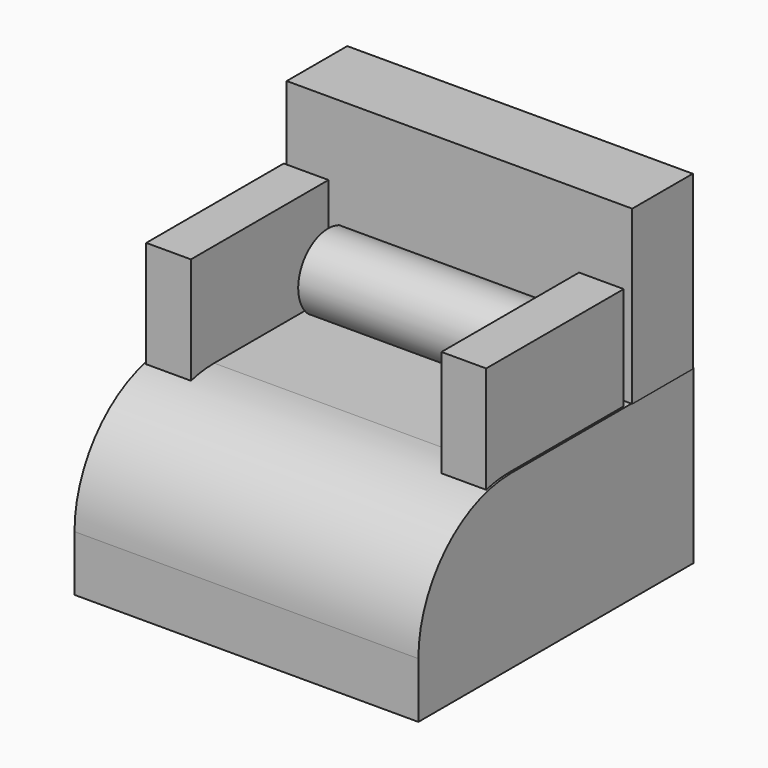
from build123d import *

# Parameters (mm, degrees)
F0_W          = 100
F0_H          = 100
F1_DEPTH      = 50
F4_DEPTH      = 50
F5_W          = 13
F5_H          = 50
F6_DEPTH      = 30
F8_R          = 10.8467438632
F9_DEPTH      = 35
F10_T4_DEPTH  = 268.9949493661
F10_T9_DEPTH  = 268.9949493661
F10_T14_DEPTH = 268.9949493661
F10_T20_DEPTH = 268.9949493661


# Not quite as in the source:
# - a fillet or chamfer that OpenCascade refuses, or shapes differently, is made with other operations: its cross-section is extruded or revolved along the edge and cut away or added


with BuildPart() as f1:
    # F0 (on Top) → F1 (new body)
    with BuildSketch(Plane.XY):
        Rectangle(F0_W, F0_H)
    extrude(amount=F1_DEPTH)

    # F3 (on offset) → F4 (join)
    with BuildSketch(Plane.XY.offset(50)):
        Polygon((49.7613176703, 49.4384859949), (-50.2386823297, 49.4384859949), (-50.2386823297, 27.4384859949), (-42.6304154098, 27.4384859949), (49.7613176703, 27.4384859949), align=None)
    extrude(amount=F4_DEPTH)

    # F5 (on offset) → F6 (join)
    with BuildSketch(Plane.XY.offset(50)):
        with Locations((-42.9296287298, 0.3518681973)):
            Rectangle(F5_W, F5_H)
    extrude(amount=F6_DEPTH)

    # F7: F1 across plane


with BuildPart() as f1_1:
    add(f1.part)
    add(f1.part.mirror(Plane.YZ))

    # F8 (on Right) → F9 (join, symmetric)
    with BuildSketch(Plane.YZ):
        with Locations((23.399380967, 57.991553098)):
            Circle(F8_R)
    extrude(amount=F9_DEPTH, both=True)

    # F10: fillet of radius 33.7989898732 on 1 edges, made by hand


with BuildPart() as f10_tool2:
    # F10_s3 → F10_t4 (new body)
    with BuildSketch(Plane.YZ.offset(-134.4974746831)):
        with BuildLine():
            ThreePointArc((-50, 16.2010101268), (-40.1005050634, 40.1005050634), (-16.2010101268, 50))
            Line((-16.2010101268, 50), (-50, 50))
            Line((-50, 50), (-50, 16.2010101268))
        make_face()
    extrude(amount=F10_T4_DEPTH)

    split(bisect_by=Plane.XZ.offset(24.6481318027), keep=Keep.TOP)


with BuildPart() as f1_2:
    add(f1_1.part)

    # F10_t1: cut F10_tool2
    add(f10_tool2.part, mode=Mode.SUBTRACT)


with BuildPart() as f10_tool7:
    # F10_s8 → F10_t9 (new body)
    with BuildSketch(Plane.YZ.offset(-134.4974746831)):
        with BuildLine():
            ThreePointArc((-50, 16.2010101268), (-40.1005050634, 40.1005050634), (-16.2010101268, 50))
            Line((-16.2010101268, 50), (-50, 50))
            Line((-50, 50), (-50, 16.2010101268))
        make_face()
    extrude(amount=F10_T9_DEPTH)

    split(bisect_by=Plane.YZ.offset(-49.4296287298), keep=Keep.BOTTOM)


with BuildPart() as f1_3:
    add(f1_2.part)

    # F10_t6: cut F10_tool7
    add(f10_tool7.part, mode=Mode.SUBTRACT)


with BuildPart() as f10_tool12:
    # F10_s13 → F10_t14 (new body)
    with BuildSketch(Plane.YZ.offset(-134.4974746831)):
        with BuildLine():
            ThreePointArc((-50, 16.2010101268), (-40.1005050634, 40.1005050634), (-16.2010101268, 50))
            Line((-16.2010101268, 50), (-50, 50))
            Line((-50, 50), (-50, 16.2010101268))
        make_face()
    extrude(amount=F10_T14_DEPTH)

    split(bisect_by=Plane.YZ.offset(-36.4296287298), keep=Keep.TOP)

    split(bisect_by=Plane.YZ.offset(36.4296287298), keep=Keep.BOTTOM)


with BuildPart() as f1_4:
    add(f1_3.part)

    # F10_t11: cut F10_tool12
    add(f10_tool12.part, mode=Mode.SUBTRACT)


with BuildPart() as f10_tool18:
    # F10_s19 → F10_t20 (new body)
    with BuildSketch(Plane.YZ.offset(-134.4974746831)):
        with BuildLine():
            ThreePointArc((-50, 16.2010101268), (-40.1005050634, 40.1005050634), (-16.2010101268, 50))
            Line((-16.2010101268, 50), (-50, 50))
            Line((-50, 50), (-50, 16.2010101268))
        make_face()
    extrude(amount=F10_T20_DEPTH)

    split(bisect_by=Plane.YZ.offset(49.4296287298), keep=Keep.TOP)


with BuildPart() as f1_5:
    add(f1_4.part)

    # F10_t17: cut F10_tool18
    add(f10_tool18.part, mode=Mode.SUBTRACT)


solid = f1_5.part
